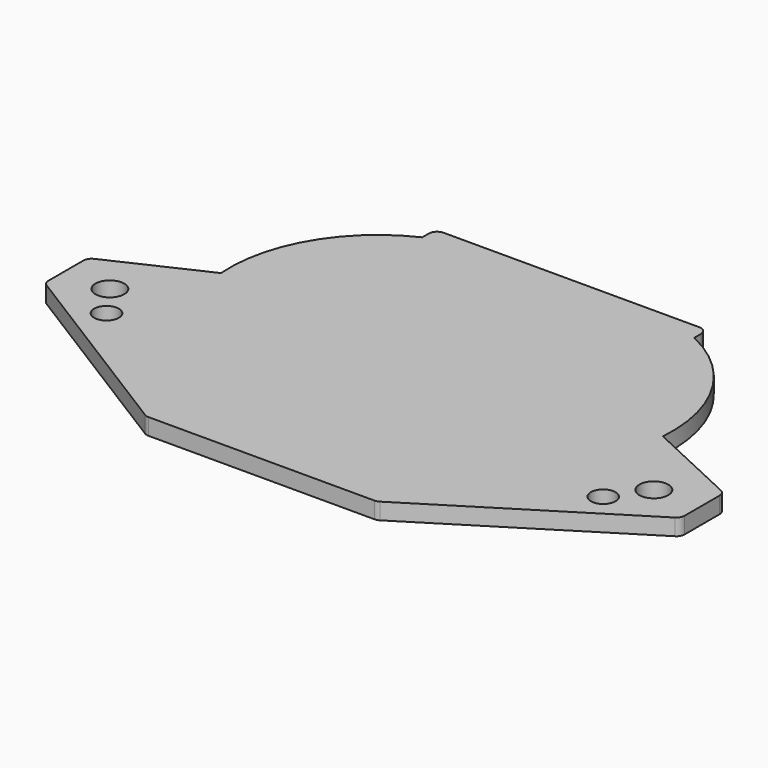
from build123d import *

# Parameters (mm, degrees)
F0_R     = 1.5
F0_R_2   = 1.75
F1_DEPTH = 2


# Not quite as in the source:
# - a feature names something its author has since deleted; it is built from what else it names


with BuildPart() as f1:
    # F0 (on Top) → F1 (new body)
    with BuildSketch(Plane.XY):
        with BuildLine():
            Line((15.5, 28.75), (0, 28.75))
            Line((0, 28.75), (-15.5, 28.75))
            ThreePointArc((-15.5, 28.75), (-16.2071067812, 28.4571067812), (-16.5, 27.75))
            Line((-16.5, 27.75), (-16.5, 26.75))
            ThreePointArc((-16.5, 26.75), (-24.4007355432, 19.5356040873), (-26.8113935571, 9.1116960654))
            Line((-26.8113935571, 9.1116960654), (-38.0160130503, 3.886896189))
            ThreePointArc((-38.0160130503, 3.886896189), (-38.4367862343, 3.5178880103), (-38.5933947885, 2.980588402))
            Line((-38.5933947885, 2.980588402), (-38.5933947885, -2.3280322858))
            ThreePointArc((-38.5933947885, -2.3280322858), (-38.4680144957, -2.812841906), (-38.1233140528, -3.1760803819))
            Line((-38.1233140528, -3.1760803819), (-14.2431738785, -18.0980480962))
            ThreePointArc((-14.2431738785, -18.0980480962), (-13.9888919701, -18.2112616959), (-13.7132546142, -18.25))
            Line((-13.7132546142, -18.25), (0, -18.25))
            Line((0, -18.25), (13.7132546142, -18.25))
            ThreePointArc((13.7132546142, -18.25), (13.9888919701, -18.2112616959), (14.2431738785, -18.0980480962))
            Line((14.2431738785, -18.0980480962), (38.1233140528, -3.1760803819))
            ThreePointArc((38.1233140528, -3.1760803819), (38.4680144957, -2.812841906), (38.5933947885, -2.3280322858))
            Line((38.5933947885, -2.3280322858), (38.5933947885, 2.980588402))
            ThreePointArc((38.5933947885, 2.980588402), (38.4367862343, 3.5178880103), (38.0160130503, 3.886896189))
            Line((38.0160130503, 3.886896189), (26.8113935571, 9.1116960654))
            ThreePointArc((26.8113935571, 9.1116960654), (24.4007355432, 19.5356040873), (16.5, 26.75))
            Line((16.5, 26.75), (16.5, 27.75))
            ThreePointArc((16.5, 27.75), (16.2071067812, 28.4571067812), (15.5, 28.75))
        make_face()
        with Locations((-30.1321178182, -4.0957602214)):
            Circle(F0_R, mode=Mode.SUBTRACT)
        with Locations((-33, 0)):
            Circle(F0_R_2, mode=Mode.SUBTRACT)
        with Locations((30.1321178182, -4.0957602214)):
            Circle(F0_R, mode=Mode.SUBTRACT)
        with Locations((33, 0)):
            Circle(F0_R_2, mode=Mode.SUBTRACT)
    extrude(amount=F1_DEPTH)


solid = f1.part
